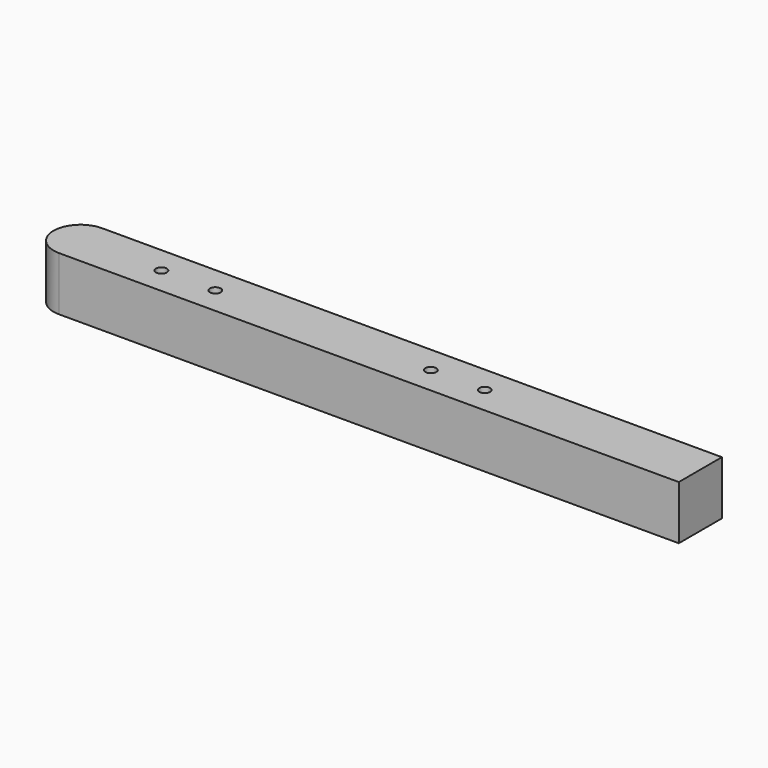
from build123d import *

# Parameters (mm, degrees)
F0_W     = 600
F0_H     = 50
F1_DEPTH = 50
F2_R     = 5
F3_DEPTH = 50.001
F4_R     = 24.99999


# Not quite as in the source:
# - a fillet or chamfer is up to 0.001 mm smaller than in the source, because OpenCascade refuses the exact size


with BuildPart() as f1:
    # F0 (on Front) → F1 (new body)
    with BuildSketch(Plane.XZ):
        with Locations((0, 10.9999733963)):
            Rectangle(F0_W, F0_H)
    extrude(amount=F1_DEPTH)

    # F2 (on face) → F3 (cut, through all)
    with BuildSketch(Plane.XY.offset(35.9999733963)):
        with Locations((50, -25)):
            Circle(F2_R)
        with Locations((-200, -25)):
            Circle(F2_R)
        with Locations((100, -25)):
            Circle(F2_R)
        with Locations((-150, -24.9278768897)):
            Circle(F2_R)
    extrude(amount=-F3_DEPTH, mode=Mode.SUBTRACT)

    # F4 (radius 25 in the source; OpenCascade refuses exactly that, so slightly less here)
    f4_edges = [f1.edges().sort_by_distance(p)[0] for p in [
        (-300, 0, 10.999973),
        (-300, -50, 10.999973),
    ]]
    fillet(f4_edges, radius=F4_R)


solid = f1.part
